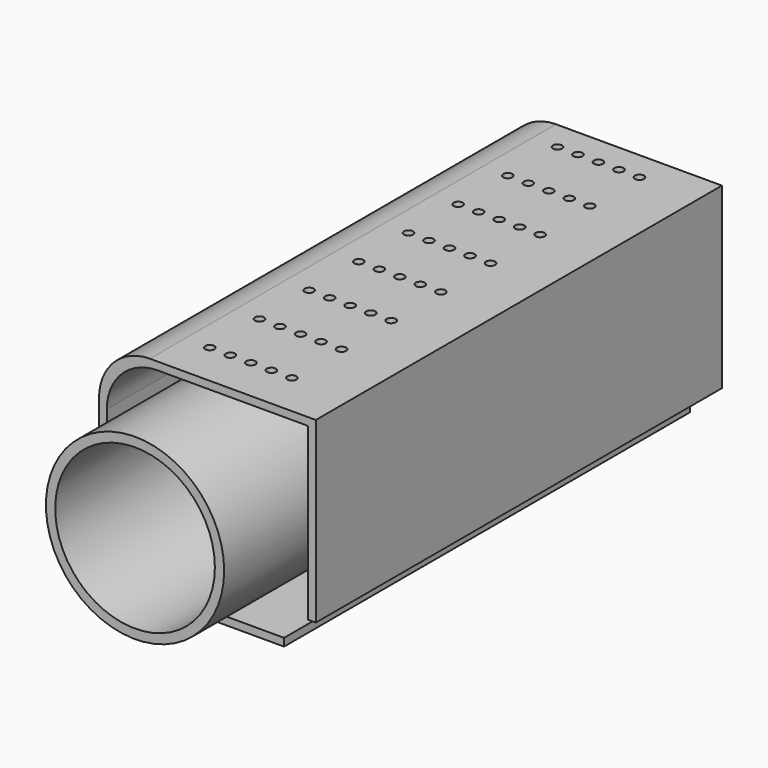
from build123d import *

# Parameters (mm, degrees)
F0_R     = 80.4081682795
F0_R_2   = 72.0317797119
F1_DEPTH = 535
F2_W     = 195.5788359046
F2_H     = 189.3626153469
F2_W_2   = 181.5788373351
F2_H_2   = 175.3626167774
F3_DEPTH = 458
F4_R     = 45.8700576851
F5_R     = 4.11720773
F6_DEPTH = 56
F7_W     = 21.679200232
F7_H     = 21.4102566242
F8_DEPTH = 939


with BuildPart() as f1:
    # F0 (on Front) → F1 (new body)
    with BuildSketch(Plane.XZ):
        Circle(F0_R)
        Circle(F0_R_2, mode=Mode.SUBTRACT)
    extrude(amount=F1_DEPTH)


with BuildPart() as f3:
    # F2 (on Front) → F3 (new body)
    with BuildSketch(Plane.XZ):
        with Locations((3.7094689906, 0.7130801678)):
            Rectangle(F2_W, F2_H)
        with Locations((3.7094689906, 0.7130801678)):
            Rectangle(F2_W_2, F2_H_2, mode=Mode.SUBTRACT)
    extrude(amount=F3_DEPTH)

    # F4
    f4_edges = [f3.edges().sort_by_distance(p)[0] for p in [
        (-87.07995, -229, 88.394389),
        (-94.079949, -229, 95.394388),
        (-87.07995, -229, -86.968228),
        (-94.079949, -229, -93.968228),
    ]]
    fillet(f4_edges, radius=F4_R)

    # F5 (on face) → F6 (cut)
    with BuildSketch(Plane.XY.offset(95.3943878412)):
        with Locations((-25.7371086627, -26.4264196157)):
            Circle(F5_R)
        with Locations((-25.7371086627, -82.4264196157)):
            Circle(F5_R)
        with Locations((-25.7371086627, -138.4264196157)):
            Circle(F5_R)
        with Locations((-25.7371086627, -194.4264196157)):
            Circle(F5_R)
        with Locations((-25.7371086627, -250.4264196157)):
            Circle(F5_R)
        with Locations((-25.7371086627, -306.4264196157)):
            Circle(F5_R)
        with Locations((-25.7371086627, -362.4264196157)):
            Circle(F5_R)
        with Locations((-25.7371086627, -418.4264196157)):
            Circle(F5_R)
        with Locations((-7.2371086627, -26.4264196157)):
            Circle(F5_R)
        with Locations((-7.2371086627, -82.4264196157)):
            Circle(F5_R)
        with Locations((-7.2371086627, -138.4264196157)):
            Circle(F5_R)
        with Locations((-7.2371086627, -194.4264196157)):
            Circle(F5_R)
        with Locations((-7.2371086627, -250.4264196157)):
            Circle(F5_R)
        with Locations((-7.2371086627, -306.4264196157)):
            Circle(F5_R)
        with Locations((-7.2371086627, -362.4264196157)):
            Circle(F5_R)
        with Locations((-7.2371086627, -418.4264196157)):
            Circle(F5_R)
        with Locations((11.2628913373, -26.4264196157)):
            Circle(F5_R)
        with Locations((11.2628913373, -82.4264196157)):
            Circle(F5_R)
        with Locations((11.2628913373, -138.4264196157)):
            Circle(F5_R)
        with Locations((11.2628913373, -194.4264196157)):
            Circle(F5_R)
        with Locations((11.2628913373, -250.4264196157)):
            Circle(F5_R)
        with Locations((11.2628913373, -306.4264196157)):
            Circle(F5_R)
        with Locations((11.2628913373, -362.4264196157)):
            Circle(F5_R)
        with Locations((11.2628913373, -418.4264196157)):
            Circle(F5_R)
        with Locations((29.7628913373, -26.4264196157)):
            Circle(F5_R)
        with Locations((29.7628913373, -82.4264196157)):
            Circle(F5_R)
        with Locations((29.7628913373, -138.4264196157)):
            Circle(F5_R)
        with Locations((29.7628913373, -194.4264196157)):
            Circle(F5_R)
        with Locations((29.7628913373, -250.4264196157)):
            Circle(F5_R)
        with Locations((29.7628913373, -306.4264196157)):
            Circle(F5_R)
        with Locations((29.7628913373, -362.4264196157)):
            Circle(F5_R)
        with Locations((29.7628913373, -418.4264196157)):
            Circle(F5_R)
        with Locations((48.2628913373, -26.4264196157)):
            Circle(F5_R)
        with Locations((48.2628913373, -82.4264196157)):
            Circle(F5_R)
        with Locations((48.2628913373, -138.4264196157)):
            Circle(F5_R)
        with Locations((48.2628913373, -194.4264196157)):
            Circle(F5_R)
        with Locations((48.2628913373, -250.4264196157)):
            Circle(F5_R)
        with Locations((48.2628913373, -306.4264196157)):
            Circle(F5_R)
        with Locations((48.2628913373, -362.4264196157)):
            Circle(F5_R)
        with Locations((48.2628913373, -418.4264196157)):
            Circle(F5_R)
    extrude(amount=-F6_DEPTH, mode=Mode.SUBTRACT)

    # F7 (on face) → F8 (cut)
    with BuildSketch(Plane(origin=(0, 0, 0), x_dir=(-1, 0, 0), z_dir=(0, 1, 0))):
        Polygon((-101.4988869429, -93.9682275057), (-72.8196874261, -93.9682275057), (-72.8196874261, -86.9682282209), (-94.4988876581, -86.9682282209), (-94.4988876581, -65.5579715967), (-101.4988869429, -65.5579715967), align=None)
        with Locations((-83.6592875421, -76.2630999088)):
            Rectangle(F7_W, F7_H)
        Polygon((-142.2729939222, -65.5579715967), (-142.2729939222, -112.1220812201), (-72.8196874261, -112.1220812201), (-72.8196874261, -93.9682275057), (-101.4988869429, -93.9682275057), (-101.4988869429, -65.5579715967), align=None)
    extrude(amount=-F8_DEPTH, mode=Mode.SUBTRACT)


solid = Compound([f1.part, f3.part])
